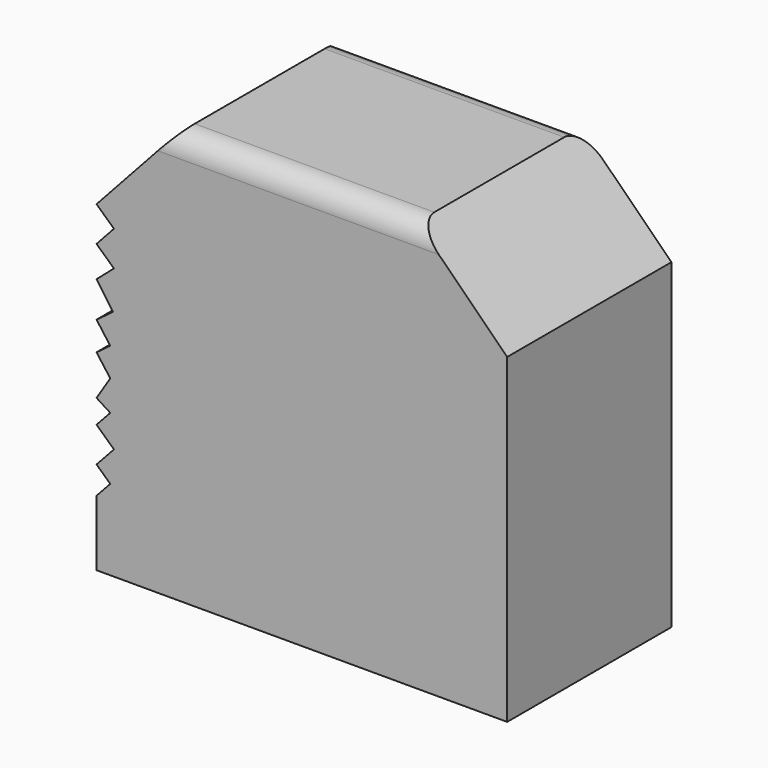
from build123d import *

# Parameters (mm, degrees)
F1_DEPTH = 152.4
F2_R     = 15.9434663659


# Not quite as in the source:
# - a feature names something its author has since deleted; it is built from what else it names


with BuildPart() as f1:
    # F0 (on Front) → F1 (new body)
    with BuildSketch(Plane.XZ):
        Polygon((-233.7148142715, -101.2738309481), (-233.7148142715, -149.9473750383), (71.0851857285, -149.9473750383), (71.0851857285, 44.3499535322), (71.0851857285, 88.5266363621), (4.2222592115, 154.8526249617), (-173.5777407885, 154.8526249617), (-233.7148142715, 89.2168954015), (-220.7819144912, 77.3674537994), (-233.7148142715, 63.2520294323), (-220.7819144912, 51.4025878302), (-233.7148142715, 40.2083918452), (-221.5843061602, 22.7510556579), (-233.7148142715, 13.7644242495), (-223.5177305101, 0), (-233.7148142715, -7.5542947057), (-223.5177305101, -21.3187189553), (-233.7148142715, -37.3470336199), (-223.5177305101, -43.8343355859), (-233.7148142715, -54.8694915965), (-220.7819144912, -66.8201937171), (-233.7148142715, -80.8160154721), (-223.5177305101, -90.2386749375), align=None)
    extrude(amount=F1_DEPTH)

    # F2
    f2_edges = [f1.edges().sort_by_distance(p)[0] for p in [
        (-84.677741, -152.4, 154.852625),
        (-84.677741, 0, 154.852625),
    ]]
    fillet(f2_edges, radius=F2_R)


solid = f1.part
